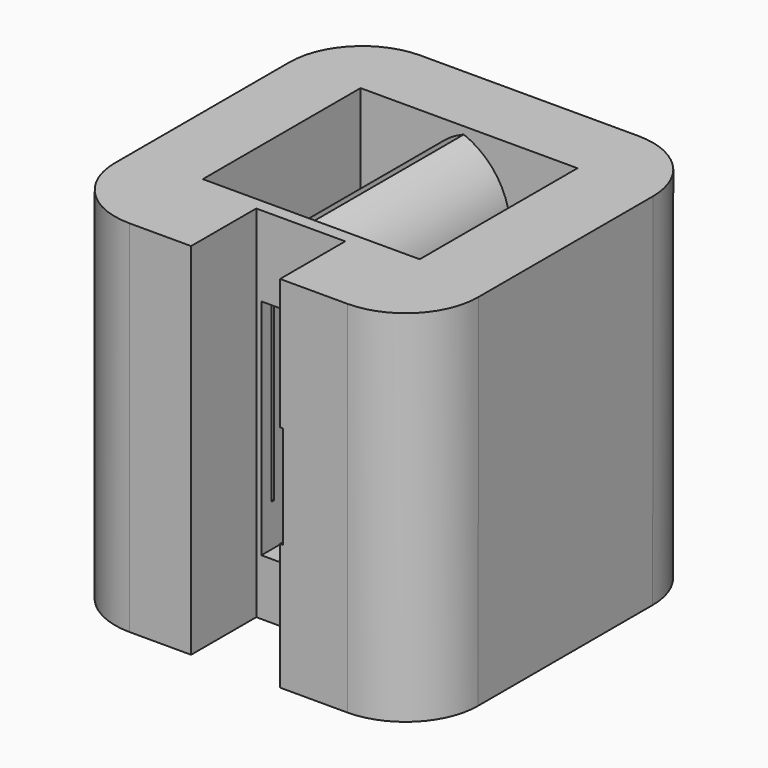
from build123d import *

# Parameters (mm, degrees)
F1_DEPTH     = 25.4
F2_W         = 15.1525349356
F2_H         = 13.7750366703
F3_DEPTH     = 18.288
F4_W         = 6.4649451524
F4_H         = 13.3289596997
F5_DEPTH     = 22.4028
F7_T1_DEPTH  = 25.1356456429
F7_T3_DEPTH  = 13.3289596997
F7_T8_DEPTH  = 50.5356473019
F7_T14_DEPTH = 50.5356473019
F8_W         = 0.189450098
F8_H         = 7.1646480085
F6_W         = 6.2150303274
F6_H         = 25.1356456429
F9_DEPTH     = 5.6896
F11_DEPTH    = 65.1764


# Not quite as in the source:
# - a fillet or chamfer that OpenCascade refuses, or shapes differently, is made with other operations: its cross-section is extruded or revolved along the edge and cut away or added


with BuildPart() as f1:
    # F0 (on Front) → F1 (new body)
    with BuildSketch(Plane.XZ):
        Polygon((0, 25.1356456429), (0, 0), (25.3690239042, 0), (25.3781564534, 25.1356456429), align=None)
    extrude(amount=F1_DEPTH)

    # F2 (on face) → F3 (cut)
    with BuildSketch(Plane.XY.offset(25.1356456429)):
        with Locations((12.512326939, -11.9383647107)):
            Rectangle(F2_W, F2_H)
    extrude(amount=-F3_DEPTH, mode=Mode.SUBTRACT)

    # F4 (on face) → F5 (join)
    with BuildSketch(Plane.XY.offset(25.1356456429)):
        with Locations((12.3413000256, -11.9561098982)):
            Rectangle(F4_W, F4_H)
    extrude(amount=-F5_DEPTH)

    # F7: fillet of radius 5.08 on 6 edges, made by hand

    # F7_s2 → F7_t1 (cut)
    with BuildSketch(Plane.XY):
        with BuildLine():
            ThreePointArc((0, -20.32), (1.4878975516, -23.9121024484), (5.08, -25.4))
            Line((5.08, -25.4), (5.08, -25.5016))
            Line((5.08, -25.5016), (-0.1016, -25.5016))
            Line((-0.1016, -25.5016), (-0.1016, -20.32))
            Line((-0.1016, -20.32), (0, -20.32))
        make_face()
        with BuildLine():
            ThreePointArc((0, -5.08), (1.4878975516, -1.4878975516), (5.08, 0))
            Line((5.08, 0), (5.08, 0.1016))
            Line((5.08, 0.1016), (-0.1016, 0.1016))
            Line((-0.1016, 0.1016), (-0.1016, -5.08))
            Line((-0.1016, -5.08), (0, -5.08))
        make_face()
    extrude(amount=F7_T1_DEPTH, mode=Mode.SUBTRACT)

    # F7_s4 → F7_t3 (cut)
    with BuildSketch(Plane.XZ.offset(5.2916300483)):
        with BuildLine():
            ThreePointArc((9.1088274494, 20.0556456429), (10.596725001, 23.6477480913), (14.1888274494, 25.1356456429))
            Line((14.1888274494, 25.1356456429), (14.1888274494, 25.2372456429))
            Line((14.1888274494, 25.2372456429), (9.0072274494, 25.2372456429))
            Line((9.0072274494, 25.2372456429), (9.0072274494, 20.0556456429))
            Line((9.0072274494, 20.0556456429), (9.1088274494, 20.0556456429))
        make_face()
        with BuildLine():
            ThreePointArc((15.5737726018, 20.0556456429), (14.0858750502, 23.6477480913), (10.4937726018, 25.1356456429))
            Line((10.4937726018, 25.1356456429), (10.4937726018, 25.2372456429))
            Line((10.4937726018, 25.2372456429), (15.6753726018, 25.2372456429))
            Line((15.6753726018, 25.2372456429), (15.6753726018, 20.0556456429))
            Line((15.6753726018, 20.0556456429), (15.5737726018, 20.0556456429))
        make_face()
    extrude(amount=F7_T3_DEPTH, mode=Mode.SUBTRACT)


with BuildPart() as f7_tool6:
    # F7_s7 → F7_t8 (new body)
    with BuildSketch(Plane(origin=(-0.0046109493, 0, -12.6907818203), x_dir=(0, 1, 0), z_dir=(0.0003633306, 0, 0.999999934))):
        with BuildLine():
            ThreePointArc((-25.4, -20.2890222297), (-23.9121024484, -23.8811246782), (-20.32, -25.3690222297))
            Line((-20.32, -25.3690222297), (-20.32, -25.4706222297))
            Line((-20.32, -25.4706222297), (-25.5016, -25.4706222297))
            Line((-25.5016, -25.4706222297), (-25.5016, -20.2890222297))
            Line((-25.5016, -20.2890222297), (-25.4, -20.2890222297))
        make_face()
    extrude(amount=F7_T8_DEPTH)

    split(bisect_by=Plane.XY.offset(25.1356456429), keep=Keep.BOTTOM)

    split(bisect_by=Plane.XY, keep=Keep.TOP)


with BuildPart() as f1_1:
    add(f1.part)

    # F7_t5: cut F7_tool6
    add(f7_tool6.part, mode=Mode.SUBTRACT)


with BuildPart() as f7_tool12:
    # F7_s13 → F7_t14 (new body)
    with BuildSketch(Plane(origin=(-0.0046109493, 0, -12.6907818203), x_dir=(0, 1, 0), z_dir=(0.0003633306, 0, 0.999999934))):
        with BuildLine():
            ThreePointArc((0, -20.2890222297), (-1.4878975516, -23.8811246782), (-5.08, -25.3690222297))
            Line((-5.08, -25.3690222297), (-5.08, -25.4706222297))
            Line((-5.08, -25.4706222297), (0.1016, -25.4706222297))
            Line((0.1016, -25.4706222297), (0.1016, -20.2890222297))
            Line((0.1016, -20.2890222297), (0, -20.2890222297))
        make_face()
    extrude(amount=F7_T14_DEPTH)

    split(bisect_by=Plane.XY.offset(25.1356456429), keep=Keep.BOTTOM)

    split(bisect_by=Plane.XY, keep=Keep.TOP)


with BuildPart() as f1_2:
    add(f1_1.part)

    # F7_t11: cut F7_tool12
    add(f7_tool12.part, mode=Mode.SUBTRACT)

    # F8 (on face) + F6 (on face) → F9 (cut)
    with BuildSketch(Plane.XZ.offset(25.4)):
        with Locations((15.687267526, 12.4311717227)):
            Rectangle(F8_W, F8_H)
    with BuildSketch(Plane.XZ.offset(25.4)):
        with Locations((12.4850273132, 12.5678228214)):
            Rectangle(F6_W, F6_H)
    extrude(amount=-F9_DEPTH, mode=Mode.SUBTRACT)

    # F10 (on face) → F11 (cut)
    with BuildSketch(Plane.XZ):
        Polygon((15.2985183522, 3.9248324286), (15.2985183522, 15.5202150633), (15.2985183522, 19.5378263631), (9.7349686548, 19.5378263631), (9.7349686548, 3.9248324286), align=None)
    extrude(amount=F11_DEPTH, mode=Mode.SUBTRACT)


solid = f1_2.part
